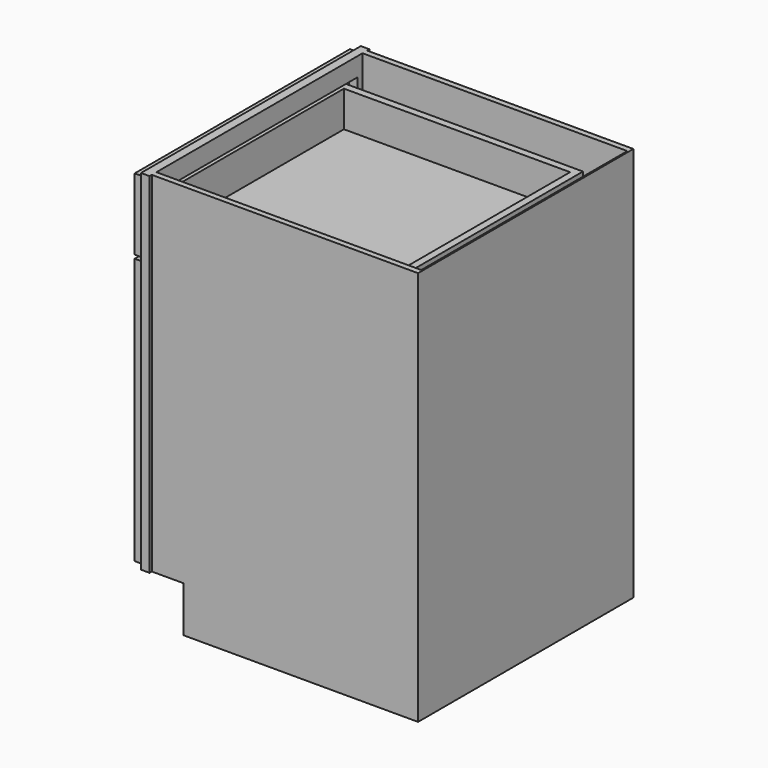
from build123d import *

# Parameters (mm, degrees)
F0_W          = 609.6
F0_H          = 876.3
F1_DEPTH      = 609.6
F2_W          = 88.9
F2_H          = 101.6
F3_DEPTH      = 609.601
F4_W          = 544.6426229508
F4_H          = 692.15
F5_DEPTH      = 19.05
F6_W          = 590.55
F6_H          = 6.35
F7_DEPTH      = 876.301
F8_W          = 587.375
F8_H          = 571.5
F9_DEPTH      = 733.425
F10_W         = 544.6426229508
F10_H         = 41.275
F11_DEPTH     = 19.05
F12_W         = 596.9
F12_H         = 590.5627
F12_W_2       = 482.6
F12_H_2       = 476.2627
F13_DEPTH     = 19.05
F14_W         = 6.35
F14_H         = 482.6
F15_DEPTH     = 476.2627
F16_SIZE      = 3.175
F17_W         = 596.9
F17_H         = 158.75
F17_W_2       = 482.6
F17_H_2       = 82.55
F18_DEPTH     = 19.05
F19_W         = 6.35
F19_H         = 482.6
F20_DEPTH     = 82.55
F21_SIZE      = 3.175
F22_W         = 504.825
F22_H         = 571.5
F23_DEPTH     = 101.6
F24_W         = 508
F24_H         = 95.25
F25_DEPTH     = 533.4
F26_T         = 15.875
F26_T3_DEPTH  = 37.249261314
F26_T5_DEPTH  = 37.249261314
F26_T7_DEPTH  = 37.249261314
F26_T9_DEPTH  = 37.249261314
F26_T11_DEPTH = 36.5125
F26_T13_DEPTH = 514.35
F26_T15_DEPTH = 114.3
F26_T17_DEPTH = 127
F26_T19_DEPTH = 539.75
F26_T21_DEPTH = 111.125
F26_T23_DEPTH = 36.5125


# Not quite as in the source:
# - a shell that OpenCascade refuses in one call is made with other operations: the cavity is built on its own and cut out


with BuildPart() as f1:
    # F0 (on Front) → F1 (new body)
    with BuildSketch(Plane.XZ):
        Rectangle(F0_W, F0_H)
    extrude(amount=-F1_DEPTH)

    # F2 (on face) → F3 (cut, through all)
    with BuildSketch(Plane.XZ):
        with Locations((-260.35, -387.35)):
            Rectangle(F2_W, F2_H)
    extrude(amount=-F3_DEPTH, mode=Mode.SUBTRACT)

    # F4 (on face) → F5 (cut)
    with BuildSketch(Plane(origin=(-304.8, 0, 0), x_dir=(0, -1, 0), z_dir=(-1, 0, 0))):
        with Locations((-304.8, 50.8)):
            Rectangle(F4_W, F4_H)
    extrude(amount=-F5_DEPTH, mode=Mode.SUBTRACT)

    # F6 (on face) → F7 (cut, through all)
    with BuildSketch(Plane.XY.offset(438.15)):
        with Locations((9.525, 606.425)):
            Rectangle(F6_W, F6_H)
        with Locations((9.525, 3.175)):
            Rectangle(F6_W, F6_H)
    extrude(amount=-F7_DEPTH, mode=Mode.SUBTRACT)

    # F8 (on face) → F9 (cut, through all)
    with BuildSketch(Plane.XY.offset(438.15)):
        with Locations((7.9375, 304.8)):
            Rectangle(F8_W, F8_H)
    extrude(amount=-F9_DEPTH, mode=Mode.SUBTRACT)

    # F10 (on face) → F11 (join, through all)
    with BuildSketch(Plane(origin=(-304.8, 0, 0), x_dir=(0, -1, 0), z_dir=(-1, 0, 0))):
        with Locations((-304.8, 265.1125)):
            Rectangle(F10_W, F10_H)
    extrude(amount=-F11_DEPTH)

    # F22 (on face) → F23 (cut)
    with BuildSketch(Plane(origin=(0, 0, -438.15), x_dir=(1, 0, 0), z_dir=(0, 0, -1))):
        with Locations((49.2125, -304.8)):
            Rectangle(F22_W, F22_H)
    extrude(amount=-F23_DEPTH, mode=Mode.SUBTRACT)


with BuildPart() as f13:
    # F12 (on face) → F13 (new body)
    with BuildSketch(Plane(origin=(-304.8, 0, 0), x_dir=(0, -1, 0), z_dir=(-1, 0, 0))):
        with Locations((-304.8, -33.33115)):
            Rectangle(F12_W, F12_H)
        with Locations((-304.8, -33.33115)):
            Rectangle(F12_W_2, F12_H_2, mode=Mode.SUBTRACT)
    extrude(amount=F13_DEPTH)

    # F14 (on face) → F15 (join, through all)
    with BuildSketch(Plane.XY.offset(-271.4625)):
        with Locations((-312.7375, 304.8)):
            Rectangle(F14_W, F14_H)
    extrude(amount=F15_DEPTH)

    # F16
    f16_edges = [f13.edges().sort_by_distance(p)[0] for p in [
        (-323.85, 546.1, -33.33115),
        (-323.85, 304.8, -271.4625),
        (-323.85, 63.5, -33.33115),
        (-323.85, 304.8, 204.8002),
    ]]
    chamfer(f16_edges, length=F16_SIZE)


with BuildPart() as f18:
    # F17 (on face) → F18 (new body)
    with BuildSketch(Plane(origin=(-304.8, 0, 0), x_dir=(0, -1, 0), z_dir=(-1, 0, 0))):
        with Locations((-304.8, 349.25)):
            Rectangle(F17_W, F17_H)
        with Locations((-304.8, 349.25)):
            Rectangle(F17_W_2, F17_H_2, mode=Mode.SUBTRACT)
    extrude(amount=F18_DEPTH)

    # F19 (on face) → F20 (join, through all)
    with BuildSketch(Plane.XY.offset(307.975)):
        with Locations((-312.7375, 304.8)):
            Rectangle(F19_W, F19_H)
    extrude(amount=F20_DEPTH)

    # F21
    f21_edges = [f18.edges().sort_by_distance(p)[0] for p in [
        (-323.85, 304.8, 307.975),
        (-323.85, 546.1, 349.25),
        (-323.85, 304.8, 390.525),
        (-323.85, 63.5, 349.25),
    ]]
    chamfer(f21_edges, length=F21_SIZE)

    # F24 (on face) → F25 (join)
    with BuildSketch(Plane.YZ.offset(-304.8)):
        with Locations((304.8, 339.725)):
            Rectangle(F24_W, F24_H)
    extrude(amount=F25_DEPTH)

    # F26: shell of thickness 15.875, made by hand


with BuildPart() as f26_core1:
    # F26_t2: copy of F18
    add(f18.part)

    # the walls: a layer under each face that stays
    f26_faces = [f26_core1.faces().sort_by_distance(p)[0] for p in [
        (-323.85, 503.7666666667, 296.3333333333),
        (-322.2625, 304.8, 306.3875),
        (-322.2625, 61.9125, 349.25),
        (-322.2625, 547.6875, 349.25),
        (-322.2625, 304.8, 392.1125),
        (-314.325, 304.8, 428.625),
        (-314.325, 603.25, 349.25),
        (-314.325, 304.8, 269.875),
        (-314.325, 6.35, 349.25),
        (-318.29375, 304.8, 307.975),
        (-318.29375, 63.5, 349.25),
        (-318.29375, 546.1, 349.25),
        (-318.29375, 304.8, 390.525),
        (-304.8, 503.7666666667, 402.1666666667),
        (-315.9125, 304.8, 349.25),
        (-38.1, 558.8, 339.725),
        (-38.1, 304.8, 292.1),
        (-38.1, 50.8, 339.725),
        (-307.18125, 63.5, 349.25),
        (-307.18125, 304.8, 390.525),
        (-307.18125, 546.1, 349.25),
        (-304.8, 304.8, 347.6625),
        (228.6, 304.8, 339.725),
        (-307.18125, 304.8, 307.975),
        (-309.5625, 304.8, 349.25),
    ]]
    thicken(f26_faces, amount=-F26_T, mode=Mode.SUBTRACT)

    # F26_s4 → F26_t3 (cut)
    with BuildSketch(Plane(origin=(4.5928978099, 4.5928978099, 4.5928978099), x_dir=(-0.7071067812, 0.7071067812, 0), z_dir=(0.5773502692, 0.5773502692, 0.5773502692))):
        Polygon((271.8908726623, 356.5892701441), (263.7152476623, 342.7036353262), (255.7777476623, 347.2863530879), (255.7777476623, 356.4517886113), align=None)
    extrude(amount=F26_T3_DEPTH, mode=Mode.SUBTRACT)

    # F26_s6 → F26_t5 (cut)
    with BuildSketch(Plane(origin=(-198.6071021901, 198.60710219, -198.6071021901), x_dir=(0.7071067812, 0.7071067812, 0), z_dir=(0.5773502692, -0.5773502692, 0.5773502692))):
        Polygon((159.161421149, 605.4574280109), (167.337046149, 591.571793193), (175.274546149, 596.1545109546), (175.274546149, 605.319946478), align=None)
    extrude(amount=F26_T5_DEPTH, mode=Mode.SUBTRACT)

    # F26_s8 → F26_t7 (cut)
    with BuildSketch(Plane(origin=(-228.2404355234, -228.2404355234, 228.2404355234), x_dir=(-0.7071067812, 0.7071067812, 0), z_dir=(0.5773502692, 0.5773502692, -0.5773502692))):
        Polygon((271.8908726623, 213.7335916339), (255.7777476623, 213.8710731668), (255.7777476623, 223.0365086901), (263.7152476623, 227.6192264518), align=None)
    extrude(amount=F26_T7_DEPTH, mode=Mode.SUBTRACT)

    # F26_s10 → F26_t9 (cut)
    with BuildSketch(Plane(origin=(-431.4404355234, 431.4404355234, 431.4404355234), x_dir=(0.7071067812, 0.7071067812, 0), z_dir=(0.5773502692, -0.5773502692, -0.5773502692))):
        Polygon((159.161421149, -35.1345662329), (175.274546149, -34.9970847), (175.274546149, -25.8316491766), (167.337046149, -21.2489314149), align=None)
    extrude(amount=F26_T9_DEPTH, mode=Mode.SUBTRACT)

    # F26_s12 → F26_t11 (cut)
    with BuildSketch(Plane.YZ.offset(-336.55)):
        Polygon((545.94125, 308.13375), (546.1, 292.1), (561.975, 292.1), (561.975, 307.975), align=None)
        Polygon((63.65875, 308.13375), (63.5, 292.1), (47.625, 292.1), (47.625, 307.975), align=None)
        Polygon((63.65875, 390.36625), (47.625, 390.525), (47.625, 406.4), (63.5, 406.4), align=None)
        Polygon((545.94125, 390.36625), (561.975, 390.525), (561.975, 406.4), (546.1, 406.4), align=None)
    extrude(amount=F26_T11_DEPTH, mode=Mode.SUBTRACT)

    # F26_s14 → F26_t13 (cut)
    with BuildSketch(Plane.XZ.offset(-561.975)):
        Polygon((-316.07125, 308.13375), (-315.9125, 292.1), (-300.0375, 292.1), (-300.0375, 307.975), align=None)
        Polygon((-316.07125, 390.36625), (-315.9125, 406.4), (-300.0375, 406.4), (-300.0375, 390.525), align=None)
        Polygon((-309.40375, 390.36625), (-309.5625, 406.4), (-325.4375, 406.4), (-325.4375, 390.525), align=None)
        Polygon((-304.95875, 308.13375), (-288.925, 307.975), (-288.925, 292.1), (-304.8, 292.1), align=None)
        Polygon((-309.40375, 308.13375), (-309.5625, 292.1), (-325.4375, 292.1), (-325.4375, 307.975), align=None)
    extrude(amount=F26_T13_DEPTH, mode=Mode.SUBTRACT)

    # F26_s16 → F26_t15 (cut)
    with BuildSketch(Plane.XY.offset(292.1)):
        Polygon((-316.07125, 63.65875), (-315.9125, 47.625), (-300.0375, 47.625), (-300.0375, 63.5), align=None)
        Polygon((-316.07125, 545.94125), (-315.9125, 561.975), (-300.0375, 561.975), (-300.0375, 546.1), align=None)
        Polygon((-309.40375, 63.65875), (-309.5625, 47.625), (-325.4375, 47.625), (-325.4375, 63.5), align=None)
        Polygon((-309.40375, 545.94125), (-309.5625, 561.975), (-325.4375, 561.975), (-325.4375, 546.1), align=None)
    extrude(amount=F26_T15_DEPTH, mode=Mode.SUBTRACT)

    # F26_s18 → F26_t17 (cut)
    with BuildSketch(Plane.XY.offset(276.225)):
        Polygon((-304.64125, 558.95875), (-320.675, 558.8), (-320.675, 542.925), (-304.8, 542.925), align=None)
        Polygon((-304.64125, 50.64125), (-320.675, 50.8), (-320.675, 66.675), (-304.8, 66.675), align=None)
    extrude(amount=F26_T17_DEPTH, mode=Mode.SUBTRACT)

    # F26_s20 → F26_t19 (cut)
    with BuildSketch(Plane.XZ.offset(-574.675)):
        Polygon((-304.64125, 291.94125), (-320.675, 292.1), (-320.675, 307.975), (-304.8, 307.975), align=None)
    extrude(amount=F26_T19_DEPTH, mode=Mode.SUBTRACT)

    # F26_s22 → F26_t21 (cut)
    with BuildSketch(Plane.XY.offset(292.1)):
        Polygon((-304.95875, 63.65875), (-304.8, 47.625), (-288.925, 47.625), (-288.925, 63.5), align=None)
        Polygon((-304.95875, 545.94125), (-304.8, 561.975), (-288.925, 561.975), (-288.925, 546.1), align=None)
    extrude(amount=F26_T21_DEPTH, mode=Mode.SUBTRACT)

    # F26_s24 → F26_t23 (cut)
    with BuildSketch(Plane.YZ.offset(-325.4375)):
        Polygon((63.65875, 308.13375), (47.625, 307.975), (47.625, 292.1), (63.5, 292.1), align=None)
        Polygon((63.65875, 390.36625), (47.625, 390.525), (47.625, 406.4), (63.5, 406.4), align=None)
        Polygon((545.94125, 390.36625), (546.1, 406.4), (561.975, 406.4), (561.975, 390.525), align=None)
        Polygon((545.94125, 308.13375), (561.975, 307.975), (561.975, 292.1), (546.1, 292.1), align=None)
    extrude(amount=F26_T23_DEPTH, mode=Mode.SUBTRACT)


with BuildPart() as f18_1:
    add(f18.part)

    # what is left inside the walls is the cavity
    f26_cavity = [f26_core1.part.solids().sort_by_distance(p)[0] for p in [
        (45.508333, 304.8, 308.13375),
    ]]
    add(f26_cavity, mode=Mode.SUBTRACT)


solid = Compound([f1.part, f13.part, f18_1.part])
